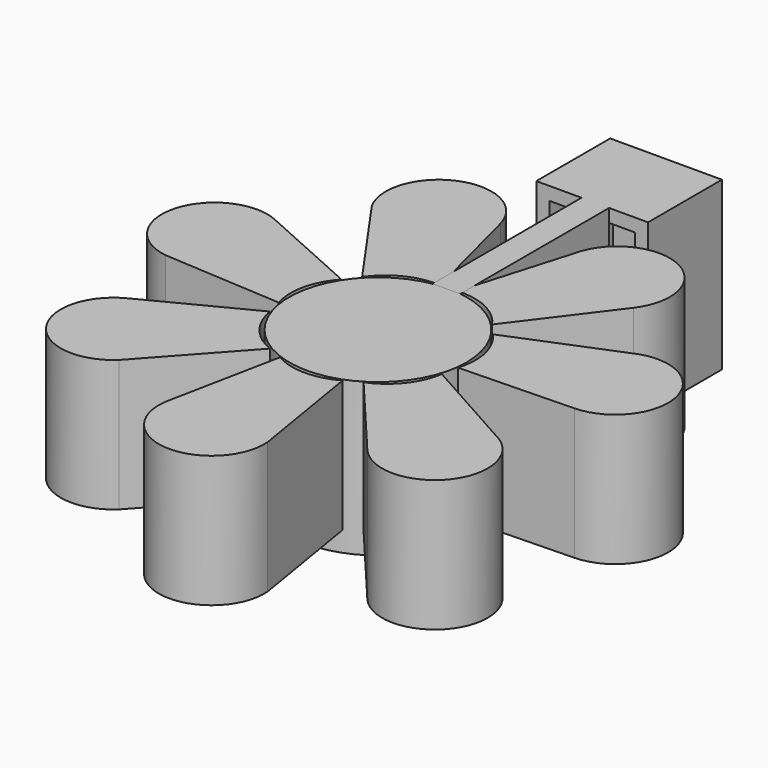
from build123d import *

# Parameters (mm, degrees)
F2_DEPTH = 25.4
F0_R     = 17.0996377698
F3_DEPTH = 29.464
F4_W     = 5.3243252914
F4_H     = 45.9828209132
F5_DEPTH = 17.78
F6_W     = 21.5624216944
F6_H     = 17.8282521665
F7_DEPTH = 32.258
F8_T     = -2.54


# Not quite as in the source:
# - a shell that OpenCascade refuses in one call is made with other operations: the cavity is built on its own and cut out


with BuildPart() as f2:
    # F1 (on Top) → F2 (new body)
    with BuildSketch(Plane.XY):
        with BuildLine():
            ThreePointArc((6.1878240667, -16.2610262632), (0.1439033076, -17.8679735925), (-5.9000174515, -16.2610262632))
            Line((-5.9000174515, -16.2610262632), (-10.2171041071, -37.8464572132))
            ThreePointArc((-10.2171041071, -37.8464572132), (-0.8065285186, -50.0180206018), (9.9292984232, -38.9976799488))
            Line((9.9292984232, -38.9976799488), (6.1878240667, -16.2610262632))
        make_face()
    extrude(amount=-F2_DEPTH)


with BuildPart() as f2b:
    # F1 (on Top) → F2, piece 2 (new body)
    with BuildSketch(Plane.XY):
        with BuildLine():
            ThreePointArc((16.5714274711, -5.3007483795), (14.0594665273, -11.0279911785), (9.034781558, -14.7514034336))
            Line((9.034781558, -14.7514034336), (23.2192915338, -31.5849337595))
            ThreePointArc((23.2192915338, -31.5849337595), (38.602800891, -31.8162951417), (36.6804302337, -16.5516176381))
            Line((36.6804302337, -16.5516176381), (16.5714274711, -5.3007483795))
        make_face()
    extrude(amount=-F2_DEPTH)


with BuildPart() as f2c:
    # F1 (on Top) → F2, piece 3 (new body)
    with BuildSketch(Plane.XY):
        with BuildLine():
            ThreePointArc((14.4764079943, 9.6511011495), (17.387964691, 4.116293523), (17.1662057784, -2.1336729446))
            Line((17.1662057784, -2.1336729446), (39.1710870626, -1.5393109697))
            ThreePointArc((39.1710870626, -1.5393109697), (48.9434338759, 10.3437494942), (35.8104499338, 18.3581503455))
            Line((35.8104499338, 18.3581503455), (14.4764079943, 9.6511011495))
        make_face()
    extrude(amount=-F2_DEPTH)


with BuildPart() as f2d:
    # F1 (on Top) → F2, piece 4 (new body)
    with BuildSketch(Plane.XY):
        with BuildLine():
            ThreePointArc((1.4803580328, 17.3354746664), (7.6229707926, 16.1609252445), (12.3711269209, 12.0907567906))
            Line((12.3711269209, 12.0907567906), (25.6262550887, 29.6654443765))
            ThreePointArc((25.6262550887, 29.6654443765), (22.4286628882, 44.7147397869), (7.9744704337, 39.443856681))
            Line((7.9744704337, 39.443856681), (1.4803580328, 17.3354746664))
        make_face()
    extrude(amount=-F2_DEPTH)


with BuildPart() as f2e:
    # F1 (on Top) → F2, piece 5 (new body)
    with BuildSketch(Plane.XY):
        with BuildLine():
            ThreePointArc((-12.6304317212, 11.9658821802), (-7.8822755929, 16.0360506342), (-1.7396628331, 17.210600056))
            Line((-1.7396628331, 17.210600056), (-7.2156696473, 38.5315150424))
            ThreePointArc((-7.2156696473, 38.5315150424), (-20.9753487157, 45.4146190056), (-25.8664479525, 30.8275344276))
            Line((-25.8664479525, 30.8275344276), (-12.6304317212, 11.9658821802))
        make_face()
    extrude(amount=-F2_DEPTH)


with BuildPart() as f2f:
    # F1 (on Top) → F2, piece 6 (new body)
    with BuildSketch(Plane.XY):
        with BuildLine():
            ThreePointArc((-17.2302487752, -2.4142636471), (-17.4520076879, 3.8357028205), (-14.5404509911, 9.370510447))
            Line((-14.5404509911, 9.370510447), (-34.6240479661, 18.3825689817))
            ThreePointArc((-34.6240479661, 18.3825689817), (-48.5844949175, 11.9163638237), (-40.2294034511, -1.0025500169))
            Line((-40.2294034511, -1.0025500169), (-17.2302487752, -2.4142636471))
        make_face()
    extrude(amount=-F2_DEPTH)


with BuildPart() as f2g:
    # F1 (on Top) → F2, piece 7 (new body)
    with BuildSketch(Plane.XY):
        with BuildLine():
            ThreePointArc((-8.8553370685, -14.9764197062), (-13.8800220378, -11.2530074511), (-16.3919829816, -5.5257646522))
            Line((-16.3919829816, -5.5257646522), (-35.9598119645, -15.6088264583))
            ThreePointArc((-35.9598119645, -15.6088264583), (-39.6085255034, -30.555156367), (-24.2987976207, -32.0776938503))
            Line((-24.2987976207, -32.0776938503), (-8.8553370685, -14.9764197062))
        make_face()
    extrude(amount=-F2_DEPTH)


with BuildPart() as f3:
    # F0 (on Top) → F3 (new body)
    with BuildSketch(Plane.XY):
        Circle(F0_R)
    extrude(amount=-F3_DEPTH)


with BuildPart() as f5:
    # F4 (on Top) → F5 (new body)
    with BuildSketch(Plane.XY):
        with Locations((-0.2835408086, 39.8713285103)):
            Rectangle(F4_W, F4_H)
    extrude(amount=-F5_DEPTH)

    # F6 (on Top) → F7 (join)
    with BuildSketch(Plane.XY):
        with Locations((-0.8888551965, 61.7097709328)):
            Rectangle(F6_W, F6_H)
    extrude(amount=-F7_DEPTH)

    # F8: a shell. OpenCascade refuses it in one call, so the cavity is built on its own and cut out:
    # the body offset inwards by the wall thickness, plus a prism from it out through each open face.
    f8_core = offset(f5.part, amount=F8_T, kind=Kind.INTERSECTION, mode=Mode.PRIVATE)
    f8_exits = [f8_core.faces().sort_by_distance(p)[0] for p in [
        (-0.893077, 55.335645, -16.179493),
    ]]
    add(f8_core, mode=Mode.SUBTRACT)
    extrude(f8_exits, amount=-F8_T, mode=Mode.SUBTRACT)


solid = Compound([f2.part, f2b.part, f2c.part, f2d.part, f2e.part, f2f.part, f2g.part, f3.part, f5.part])
